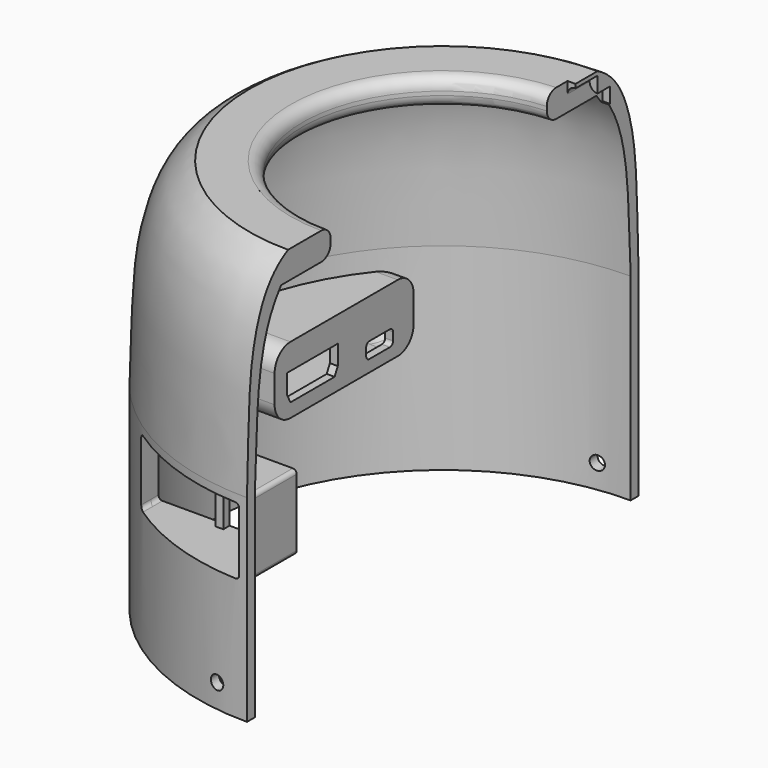
from build123d import *

# Parameters (mm, degrees)
F1_ANGLE_BACK = 90
F1_ANGLE      = 180
F3_DEPTH      = 49
F4_DEPTH      = 42
F5_DEPTH      = 53
F8_DEPTH      = 25
F10_DEPTH     = 2
F11_W         = 1
F11_H         = 5
F11_W_2       = 14
F11_H_2       = 2
F12_DEPTH     = 2
F14_W         = 2
F14_H         = 17
F15_REACH     = 40.3462351599
F16_REACH     = 57.7072649741
F17_DEPTH     = 2
F18_R         = 1.75
F19_DEPTH     = 62.5


with BuildPart() as f1:
    # F0 (on Front) → F1 (revolve)
    with BuildSketch(Plane.XZ, mode=Mode.PRIVATE) as f1_sk:
        with BuildLine():
            ThreePointArc((-35.5, 47), (-36.3786796564, 49.1213203436), (-38.5, 50))
            Line((-38.5, 50), (-49, 50))
            add(Edge.make_bspline(
                [(-49, 50), (-50.0905438599, 49.4592544488), (-53.0493875637, 47.4989733534), (-57.4486951492, 41.931344871), (-61.5763053799, 28.0443008729), (-61.4881986154, 14.5014666819), (-62, 0)],
                knots=[0, 0, 0, 0, 0.1531073754, 0.3436852098, 0.6019385566, 1, 1, 1, 1], degree=3))
            Line((-62, 0), (-62, -50))
            Line((-62, -50), (-59.5, -50))
            Line((-59.5, -50), (-59.5, 0))
            add(Edge.make_bspline(
                [(-51.1955396277, 43), (-59.7999691963, 32.3488041759), (-58.4857873619, 15.5563373119), (-59.5, 0)],
                knots=[0, 0, 0, 0, 43.7945665817, 43.7945665817, 43.7945665817, 43.7945665817], degree=3))
            Line((-51.1955396277, 43), (-38.5, 43))
            ThreePointArc((-38.5, 43), (-36.3786796564, 43.8786796564), (-35.5, 46))
            Line((-35.5, 46), (-35.5, 47))
        make_face()
    revolve(f1_sk.sketch.rotate(Axis((0, 0, -47.5967168808), (0, 0, 1)), -F1_ANGLE_BACK), axis=Axis((0, 0, -47.5967168808), (0, 0, 1)), revolution_arc=F1_ANGLE)

    # F2 (on Front) → F3 (cut)
    with BuildSketch(Plane.XZ):
        with BuildLine():
            ThreePointArc((0, 45), (1.4142135624, 45.5857864376), (2, 47))
            ThreePointArc((2, 47), (1.4142135624, 48.4142135624), (0, 49))
            ThreePointArc((0, 49), (-1.3909130574, 48.4371363424), (-1.998931704, 47.0653608667))
            Line((-1.998931704, 47.0653608667), (-1.998931704, 46.9346391333))
            ThreePointArc((-1.998931704, 46.9346391333), (-1.3909130574, 45.5628636576), (0, 45))
        make_face()
    extrude(amount=-F3_DEPTH, mode=Mode.SUBTRACT)

    # F2 (on Front) → F4 (cut)
    with BuildSketch(Plane.XZ):
        with BuildLine():
            ThreePointArc((-1.998931704, 47.0653608667), (-1.3909130574, 48.4371363424), (0, 49))
            Line((0, 49), (0, 50.3604523001))
            Line((0, 50.3604523001), (-1.998931704, 50.3604523001))
            Line((-1.998931704, 50.3604523001), (-1.998931704, 47.0653608667))
        make_face()
    extrude(amount=-F4_DEPTH, mode=Mode.SUBTRACT)

    # F2 (on Front) → F5 (cut)
    with BuildSketch(Plane.XZ):
        with BuildLine():
            Line((0, 41.0653608667), (0, 45))
            ThreePointArc((0, 45), (-1.3909130574, 45.5628636576), (-1.998931704, 46.9346391333))
            Line((-1.998931704, 46.9346391333), (-1.998931704, 41.0653608667))
            Line((-1.998931704, 41.0653608667), (0, 41.0653608667))
        make_face()
    extrude(amount=-F5_DEPTH, mode=Mode.SUBTRACT)

    # F7 (on offset) → F8 (cut)
    with BuildSketch(Plane.YZ.offset(-41)):
        with BuildLine():
            Line((36, -6), (4, -6))
            ThreePointArc((4, -6), (0.4644660941, -7.4644660941), (-1, -11))
            Line((-1, -11), (-1, -16))
            ThreePointArc((-1, -16), (0.4644660941, -19.5355339059), (4, -21))
            Line((4, -21), (36, -21))
            ThreePointArc((36, -21), (39.5355339059, -19.5355339059), (41, -16))
            Line((41, -16), (41, -11))
            ThreePointArc((41, -11), (39.5355339059, -7.4644660941), (36, -6))
        make_face()
    extrude(amount=-F8_DEPTH, mode=Mode.SUBTRACT)

    # F7 (on offset) → F9 (join, up to the next surface of F1)
    with BuildSketch(Plane.YZ.offset(-41)):
        with BuildLine():
            Line((42, -17), (42, -10))
            ThreePointArc((42, -10), (40.5355339059, -6.4644660941), (37, -5))
            Line((37, -5), (3, -5))
            ThreePointArc((3, -5), (-0.5355339059, -6.4644660941), (-2, -10))
            Line((-2, -10), (-2, -17))
            ThreePointArc((-2, -17), (-0.5355339059, -20.5355339059), (3, -22))
            Line((3, -22), (37, -22))
            ThreePointArc((37, -22), (40.5355339059, -20.5355339059), (42, -17))
        make_face()
        with BuildLine():
            ThreePointArc((-1, -11), (0.4644660941, -7.4644660941), (4, -6))
            Line((4, -6), (36, -6))
            ThreePointArc((36, -6), (39.5355339059, -7.4644660941), (41, -11))
            Line((41, -11), (41, -16))
            ThreePointArc((41, -16), (39.5355339059, -19.5355339059), (36, -21))
            Line((36, -21), (4, -21))
            ThreePointArc((4, -21), (0.4644660941, -19.5355339059), (-1, -16))
            Line((-1, -16), (-1, -11))
        make_face(mode=Mode.SUBTRACT)
    extrude(until=Until.NEXT, dir=(-1, 0, 0))

    # F7 (on offset) → F10 (join)
    with BuildSketch(Plane.YZ.offset(-41)):
        with BuildLine():
            Line((36, -6), (4, -6))
            ThreePointArc((4, -6), (0.4644660941, -7.4644660941), (-1, -11))
            Line((-1, -11), (-1, -16))
            ThreePointArc((-1, -16), (0.4644660941, -19.5355339059), (4, -21))
            Line((4, -21), (36, -21))
            ThreePointArc((36, -21), (39.5355339059, -19.5355339059), (41, -16))
            Line((41, -16), (41, -11))
            ThreePointArc((41, -11), (39.5355339059, -7.4644660941), (36, -6))
        make_face()
    extrude(amount=-F10_DEPTH)

    # F11 (on offset) → F12 (cut)
    with BuildSketch(Plane.YZ.offset(-41)):
        with BuildLine():
            Line((34.5, -15), (28, -15))
            ThreePointArc((28, -15), (27.2928932188, -15.2928932188), (27, -16))
            Line((27, -16), (27, -18))
            ThreePointArc((27, -18), (27.2928932188, -18.7071067812), (28, -19))
            Line((28, -19), (34.5, -19))
            ThreePointArc((34.5, -19), (35.2071067812, -18.7071067812), (35.5, -18))
            Line((35.5, -18), (35.5, -16))
            ThreePointArc((35.5, -16), (35.2071067812, -15.2928932188), (34.5, -15))
        make_face()
        with Locations((2.5, -14)):
            Rectangle(F11_W, F11_H)
        with Locations((10, -14)):
            Rectangle(F11_W_2, F11_H)
        Polygon((3, -16.5), (2, -16.5), (3, -18.5), align=None)
        with Locations((17.5, -14)):
            Rectangle(F11_W, F11_H)
        with Locations((10, -17.5)):
            Rectangle(F11_W_2, F11_H_2)
        Polygon((18, -16.5), (17, -16.5), (17, -18.5), align=None)
    extrude(amount=-F12_DEPTH, mode=Mode.SUBTRACT)

    f15_end = f1.faces().sort_by_distance((-62, 0, -25))[0]
    # F14 (on offset) → F15 (cut, up to a face of the model that its end follows)
    with BuildSketch(Plane.XZ.offset(45)):
        with Locations((-19, -10.5)):
            Rectangle(F14_W, F14_H)
        with BuildLine():
            Line((-20, -2), (-35, -2))
            ThreePointArc((-35, -2), (-35.7071067812, -2.2928932188), (-36, -3))
            Line((-36, -3), (-36, -18))
            ThreePointArc((-36, -18), (-35.7071067812, -18.7071067812), (-35, -19))
            Line((-35, -19), (-20, -19))
            Line((-20, -19), (-20, -2))
        make_face()
        with BuildLine():
            Line((-3, -2), (-18, -2))
            Line((-18, -2), (-18, -19))
            Line((-18, -19), (-3, -19))
            ThreePointArc((-3, -19), (-2.2928932188, -18.7071067812), (-2, -18))
            Line((-2, -18), (-2, -3))
            ThreePointArc((-2, -3), (-2.2928932188, -2.2928932188), (-3, -2))
        make_face()
    f15_long = extrude(amount=F15_REACH, mode=Mode.PRIVATE)
    add(split(f15_long, bisect_by=f15_end, keep=Keep.BOTTOM, mode=Mode.PRIVATE), mode=Mode.SUBTRACT)

    f16_end = f1.faces().sort_by_distance((-62, 0, -25))[0]
    # F14 (on offset) → F16 (join, up to a face of the model that its end follows)
    with BuildSketch(Plane.XZ.offset(45)):
        with BuildLine():
            ThreePointArc((-1, -2), (-1.2928932188, -1.2928932188), (-2, -1))
            Line((-2, -1), (-36, -1))
            ThreePointArc((-36, -1), (-36.7071067812, -1.2928932188), (-37, -2))
            Line((-37, -2), (-37, -19))
            ThreePointArc((-37, -19), (-36.7071067812, -19.7071067812), (-36, -20))
            Line((-36, -20), (-2, -20))
            ThreePointArc((-2, -20), (-1.2928932188, -19.7071067812), (-1, -19))
            Line((-1, -19), (-1, -2))
        make_face()
        with BuildLine():
            ThreePointArc((-36, -3), (-35.7071067812, -2.2928932188), (-35, -2))
            Line((-35, -2), (-20, -2))
            Line((-20, -2), (-18, -2))
            Line((-18, -2), (-3, -2))
            ThreePointArc((-3, -2), (-2.2928932188, -2.2928932188), (-2, -3))
            Line((-2, -3), (-2, -18))
            ThreePointArc((-2, -18), (-2.2928932188, -18.7071067812), (-3, -19))
            Line((-3, -19), (-18, -19))
            Line((-18, -19), (-20, -19))
            Line((-20, -19), (-35, -19))
            ThreePointArc((-35, -19), (-35.7071067812, -18.7071067812), (-36, -18))
            Line((-36, -18), (-36, -3))
        make_face(mode=Mode.SUBTRACT)
    f16_long = extrude(amount=F16_REACH, mode=Mode.PRIVATE)
    add(split(f16_long, bisect_by=f16_end, keep=Keep.BOTTOM, mode=Mode.PRIVATE))

    # F14 (on offset) → F17 (join)
    with BuildSketch(Plane.XZ.offset(45)):
        with Locations((-19, -10.5)):
            Rectangle(F14_W, F14_H)
    extrude(amount=F17_DEPTH)

    # F18 (on Front) → F19 (cut, symmetric)
    with BuildSketch(Plane.XZ):
        with Locations((-8, -44)):
            Circle(F18_R)
    extrude(amount=F19_DEPTH, both=True, mode=Mode.SUBTRACT)


solid = f1.part
